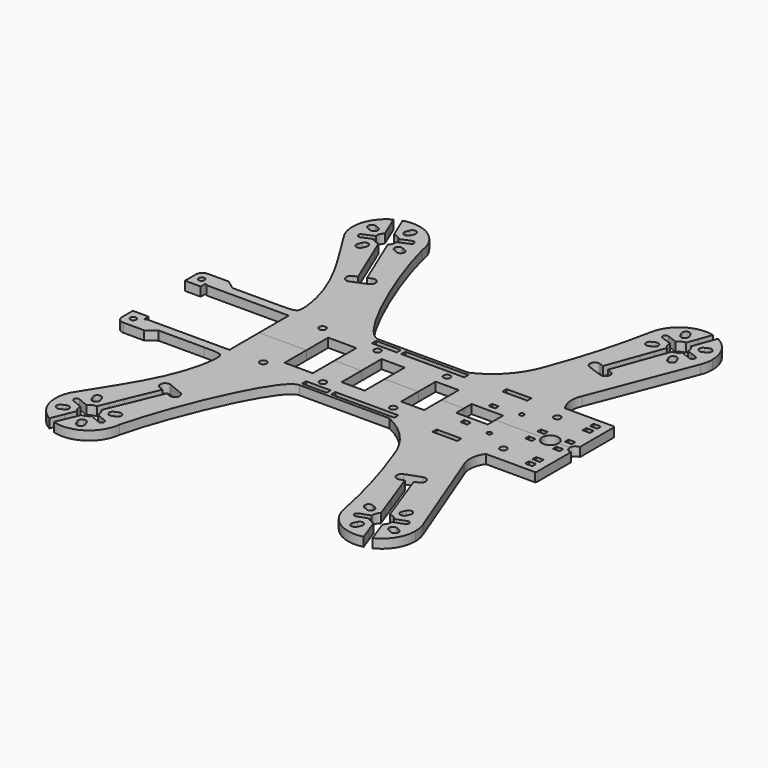
from build123d import *
from build123d import SkipClean  # not in build123d's __all__

# Parameters (mm, degrees)
F0_R     = 1.3067583218
F0_R_2   = 1.5
F0_W     = 11
F0_H     = 2.3
F0_W_2   = 28
F0_W_3   = 3
F0_H_2   = 2
F0_R_3   = 1
F0_W_4   = 7
F0_W_5   = 3.27
F0_H_3   = 1.9745780493
F1_DEPTH = 4


# Not quite as in the source:
# - ends of sketch curves that miss each other by under 0.0002 mm in the source are joined
# - a feature names something its author has since deleted; it is built from what else it names


with BuildPart() as f1:
    # F0 (on Top) → F1 (new body)
    with BuildSketch(Plane.XY):
        with BuildLine():
            Line((23.807834385, 10.9809627828), (66.6183753957, 10.9809627828))
            ThreePointArc((66.6183753957, 10.9809627828), (64.6130521178, 16.2439737053), (65.5746503361, 21.793382168))
            Line((65.5746503361, 21.793382168), (82.7334265347, 66.1261316559))
            ThreePointArc((82.7334265347, 66.1261316559), (75.7149263237, 58.2772137012), (65.2621276006, 57.0107788924))
            Line((65.2621276006, 57.0107788924), (60.1318261331, 42.9153893322))
            Line((60.1318261331, 42.9153893322), (61.889296675, 42.2757224637))
            ThreePointArc((61.889296675, 42.2757224637), (63.1828697728, 39.5016463539), (60.408793663, 38.2080732561))
            Line((60.408793663, 38.2080732561), (53.8309452016, 40.6022139409))
            ThreePointArc((53.8309452016, 40.6022139409), (52.5374310433, 43.3761636546), (55.311380757, 44.6696778129))
            Line((55.311380757, 44.6696778129), (57.0693637919, 44.0301103067))
            Line((57.0693637919, 44.0301103067), (62.1996652593, 58.1254998669))
            ThreePointArc((62.1996652593, 58.1254998669), (55.4315651943, 64.8791097008), (54.1477200077, 74.3538216129))
            ThreePointArc((54.1477200077, 74.3538216129), (49.0043825672, 52.7428496664), (42.0475143877, 31.6456931368))
            ThreePointArc((42.0475143877, 31.6456931368), (35.1236653457, 19.3750412413), (23.807834385, 10.9809627828))
        make_face()
        with BuildLine():
            Line((81.307834385, -10.9840372172), (86.307834385, -10.9840372172))
            ThreePointArc((86.307834385, -10.9840372172), (87.040067432, -9.2162702643), (88.807834385, -8.4840372172))
            Line((88.807834385, -8.4840372172), (88.807834385, 10.2602147337))
            Line((88.807834385, 10.2602147337), (88.807834385, 10.2855553205))
            ThreePointArc((88.807834385, 10.2855553205), (88.6955077799, 10.6869222269), (88.4001219115, 10.9809627828))
            Line((88.4001219115, 10.9809627828), (66.6183753957, 10.9809627828))
            Line((66.6183753957, 10.9809627828), (23.807834385, 10.9809627828))
            Line((23.807834385, 10.9809627828), (-16.192165615, 10.9809627828))
            add(Edge.make_bspline(
                [(-46.3442459805, 73.1007904778), (-41.173171252, 51.9413948059), (-24.192165615, 10.9809627828), (-16.192165615, 10.9809627828)],
                knots=[0, 0, 0, 0, 69.0508576574, 69.0508576574, 69.0508576574, 69.0508576574], degree=3))
            ThreePointArc((-46.3442459805, 73.1007904778), (-46.2810054236, 72.3094979368), (-46.259905361, 71.5159627828))
            ThreePointArc((-46.259905361, 71.5159627828), (-48.3312280894, 63.9285599164), (-53.970550806, 58.4461243811))
            Line((-53.970550806, 58.4461243811), (-48.1929196847, 44.603473673))
            Line((-48.1929196847, 44.603473673), (-46.4646633816, 45.3248114871))
            ThreePointArc((-46.4646633816, 45.3248114871), (-43.6333050022, 44.1609667989), (-44.7971496904, 41.3296084195))
            Line((-44.7971496904, 41.3296084195), (-51.2570532871, 38.6333805908))
            ThreePointArc((-51.2570532871, 38.6333805908), (-54.087935927, 39.7970297238), (-52.9242867941, 42.6279123637))
            Line((-52.9242867941, 42.6279123637), (-51.200432983, 43.3480286655))
            Line((-51.200432983, 43.3480286655), (-56.9780641043, 57.1906793736))
            ThreePointArc((-56.9780641043, 57.1906793736), (-65.7737180803, 57.3039336067), (-72.9794719714, 62.3490764437))
            add(Edge.make_bspline(
                [(-72.9794719714, 62.3490764437), (-63.3735946314, 46.7592850211), (-53.3038261444, 32.6817020671), (-51.3139774001, 14.7110713705)],
                knots=[3.2172773319, 3.2172773319, 3.2172773319, 3.2172773319, 55.6902315894, 55.6902315894, 55.6902315894, 55.6902315894], degree=3))
            add(Edge.make_bspline(
                [(-59.884751521, 9.4825), (-49.8880036175, 9.3324426562), (-51.4223264341, 10.2774120803), (-51.3139774001, 14.7110713705)],
                knots=[0, 0, 0, 0, 10.0397274668, 10.0397274668, 10.0397274668, 10.0397274668], degree=3))
            Line((-59.884751521, 9.4825), (-79.884751521, 9.4825))
            Line((-79.884751521, 9.4825), (-83.984751521, 12.4825))
            Line((-83.984751521, 12.4825), (-93.184751521, 12.4825))
            Line((-93.184751521, 12.4825), (-93.2316647449, 12.4825))
            ThreePointArc((-93.2316647449, 12.4825), (-95.3130075003, 11.6107559793), (-96.184751521, 9.5294132239))
            Line((-96.184751521, 9.5294132239), (-96.184751521, 9.4825))
            Line((-96.184751521, 9.4825), (-96.184751521, 5.4825))
            Line((-96.184751521, 5.4825), (-89.184751521, 5.4825))
            ThreePointArc((-89.184751521, 5.4825), (-88.684751521, 5.9825), (-88.184751521, 5.4825))
            Line((-88.184751521, 5.4825), (-51.684751521, 5.4825))
            Line((-51.684751521, 5.4825), (-51.684751521, -10.9840372172))
            Line((-51.684751521, -10.9840372172), (-30.662165615, -10.9840372172))
            Line((-30.662165615, -10.9840372172), (-30.662165615, 1.1159627828))
            Line((-30.662165615, 1.1159627828), (-18.162165615, 1.1159627828))
            Line((-18.162165615, 1.1159627828), (-18.162165615, -10.9840372172))
            Line((-18.162165615, -10.9840372172), (-6.162165615, -10.9840372172))
            Line((-6.162165615, -10.9840372172), (-6.162165615, 0.1159627828))
            Line((-6.162165615, 0.1159627828), (4.087834385, 0.1159627828))
            Line((4.087834385, 0.1159627828), (4.087834385, -10.9840372172))
            Line((4.087834385, -10.9840372172), (19.087834385, -10.9840372172))
            Line((19.087834385, -10.9840372172), (19.087834385, -1.3840372172))
            Line((19.087834385, -1.3840372172), (29.307834385, -1.3840372172))
            Line((29.307834385, -1.3840372172), (29.307834385, -10.9840372172))
            Line((29.307834385, -10.9840372172), (39.307834385, -10.9840372172))
            Line((39.307834385, -10.9840372172), (39.307834385, -6.7155264844))
            Line((39.307834385, -6.7155264844), (53.307834385, -6.7155264844))
            Line((53.307834385, -6.7155264844), (53.307834385, -10.9840372172))
            Line((53.307834385, -10.9840372172), (74.017834385, -10.9840372172))
            ThreePointArc((74.017834385, -10.9840372172), (77.662834385, -7.3390372172), (81.307834385, -10.9840372172))
        make_face()
        with Locations((-92.384751521, 7.9825)):
            Circle(F0_R, mode=Mode.SUBTRACT)
        with Locations((-36.662165615, 5.4809627828)):
            Circle(F0_R_2, mode=Mode.SUBTRACT)
        with Locations((-11.184751521, 4.1809627828)):
            Circle(F0_R_2, mode=Mode.SUBTRACT)
        with Locations((-10.692165615, 8.4309627828)):
            Rectangle(F0_W, F0_H, mode=Mode.SUBTRACT)
        with Locations((10.807834385, 8.4309627828)):
            Rectangle(F0_W_2, F0_H, mode=Mode.SUBTRACT)
        with Locations((19.807834385, 3.9809627828)):
            Circle(F0_R_2, mode=Mode.SUBTRACT)
        with Locations((46.307834385, -3.2155264844)):
            Rectangle(F0_W_3, F0_H_2, mode=Mode.SUBTRACT)
        with Locations((57.807834385, -2.0190372172)):
            Circle(F0_R_3, mode=Mode.SUBTRACT)
        with Locations((71.517834385, -7.6190372172)):
            Rectangle(F0_W_3, F0_H_2, mode=Mode.SUBTRACT)
        with Locations((83.807834385, -7.6190372172)):
            Rectangle(F0_W_3, F0_H_2, mode=Mode.SUBTRACT)
        with Locations((47.307834385, 8.4309627828)):
            Rectangle(F0_W, F0_H, mode=Mode.SUBTRACT)
        with Locations((68.807834385, 3.9809627828)):
            Circle(F0_R_2, mode=Mode.SUBTRACT)
        Polygon((81.687834385, 5.9782518074), (81.687834385, 8.0809627828), (84.957834385, 8.0809627828), (84.957834385, 5.9782518074), (84.957834385, 4.0036737581), (84.957834385, 1.9009627828), (81.687834385, 1.9009627828), (81.687834385, 4.0036737581), align=None, mode=Mode.SUBTRACT)
        with Locations((-92.684751521, 4.4825)):
            Rectangle(F0_W_4, F0_H_2)
        with BuildLine():
            ThreePointArc((65.2621276006, 57.0107788924), (75.7149263237, 58.2772137012), (82.7334265347, 66.1261316559))
            ThreePointArc((82.7334265347, 66.1261316559), (83.486270311, 68.7744458556), (83.7400946391, 71.5159627828))
            ThreePointArc((83.7400946391, 71.5159627828), (81.4895193699, 79.3993162722), (75.416202451, 84.9063275201))
            Line((75.416202451, 84.9063275201), (73.3649143135, 79.271103595))
            Line((73.3649143135, 79.271103595), (71.6900636377, 74.6700149294))
            ThreePointArc((71.6900636377, 74.6700149294), (72.7174356247, 73.2394210952), (73.0804554083, 71.5159627828))
            ThreePointArc((73.0804554083, 71.5159627828), (73.0780687132, 71.3731720581), (73.0709112943, 71.2305408599))
            Line((73.0709112943, 71.2305408599), (77.6719999599, 69.5556901841))
            ThreePointArc((77.6719999599, 69.5556901841), (78.383174195, 68.0304258767), (76.8579098876, 67.3192516416))
            Line((76.8579098876, 67.3192516416), (72.256821222, 68.9941023174))
            ThreePointArc((72.256821222, 68.9941023174), (70.8217224071, 67.7477343604), (68.9880509133, 67.2471441627))
            Line((68.9880509133, 67.2471441627), (67.3132002375, 62.646055497))
            Line((67.3132002375, 62.646055497), (65.2621276006, 57.0107788924))
        make_face()
        with BuildLine():
            Line((71.6865255454, 61.4383570551), (70.968074214, 62.9790809073))
            ThreePointArc((70.968074214, 62.9790809073), (70.9135396748, 64.2404537845), (71.7658205961, 65.1719325992))
            ThreePointArc((71.7658205961, 65.1719325992), (71.7659371457, 65.1719871288), (71.7660536995, 65.1720416494))
            ThreePointArc((71.7660536995, 65.1720416494), (73.0273231534, 65.2262270051), (73.9585485766, 64.3738448825))
            Line((73.9585485766, 64.3738448825), (74.6936236673, 62.7974712634))
            ThreePointArc((74.6936236673, 62.7974712634), (74.7249665763, 61.5535139642), (73.8793778852, 60.6406109543))
            ThreePointArc((73.8793778852, 60.6406109543), (72.6180046911, 60.5860759997), (71.6865255454, 61.4383570551))
        make_face(mode=Mode.SUBTRACT)
        with BuildLine():
            Line((78.8853157659, 74.3943123226), (77.3445925279, 73.6758612777))
            ThreePointArc((77.3445925279, 73.6758612777), (76.0832108836, 73.6215228577), (75.1518645475, 74.4739489944))
            ThreePointArc((75.1518645475, 74.4739489944), (75.0975261275, 75.7353306387), (75.9499522642, 76.6666769749))
            Line((75.9499522642, 76.6666769749), (77.4906755022, 77.3851280199))
            ThreePointArc((77.4906755022, 77.3851280199), (78.7520571465, 77.4394664398), (79.6834034826, 76.5870403031))
            ThreePointArc((79.6834034826, 76.5870403031), (79.7377419026, 75.3256586588), (78.8853157659, 74.3943123226))
        make_face(mode=Mode.SUBTRACT)
        with BuildLine():
            ThreePointArc((72.35375667, 86.0210939936), (60.7509970609, 84.0881451163), (54.1477200077, 74.3538216129))
            ThreePointArc((54.1477200077, 74.3538216129), (55.4315651943, 64.8791097008), (62.1996652593, 58.1254998669))
            Line((62.1996652593, 58.1254998669), (64.2507544565, 63.7608219705))
            Line((64.2507544565, 63.7608219705), (65.9256051324, 68.3619106361))
            ThreePointArc((65.9256051324, 68.3619106361), (64.8428191889, 69.9241258241), (64.5447574757, 71.8013847056))
            Line((64.5447574757, 71.8013847056), (59.9436688101, 73.4762353814))
            ThreePointArc((59.9436688101, 73.4762353814), (59.232494575, 75.0014996888), (60.7577588824, 75.7126739239))
            Line((60.7577588824, 75.7126739239), (65.358847548, 74.0378232481))
            ThreePointArc((65.358847548, 74.0378232481), (66.7939463629, 75.2841912051), (68.6276178567, 75.7847814029))
            Line((68.6276178567, 75.7847814029), (70.3024685325, 80.3858700685))
            Line((70.3024685325, 80.3858700685), (72.35375667, 86.0210939936))
        make_face()
        with BuildLine():
            ThreePointArc((57.9321409406, 66.4445436419), (57.8778025206, 67.7059252862), (58.7302286573, 68.6372716224))
            Line((58.7302286573, 68.6372716224), (60.2709518953, 69.3557226673))
            ThreePointArc((60.2709518953, 69.3557226673), (61.5323335396, 69.4100610873), (62.4636798757, 68.5576349506))
            ThreePointArc((62.4636798757, 68.5576349506), (62.5180182957, 67.2962533063), (61.665592159, 66.3649069701))
            Line((61.665592159, 66.3649069701), (60.124868921, 65.6464559251))
            ThreePointArc((60.124868921, 65.6464559251), (58.8634872767, 65.5921175051), (57.9321409406, 66.4445436419))
        make_face(mode=Mode.SUBTRACT)
        with BuildLine():
            ThreePointArc((65.8495068393, 77.8601166777), (64.588125195, 77.8057782577), (63.6567788588, 78.6582043944))
            Line((63.6567788588, 78.6582043944), (62.9383275274, 80.1989282467))
            ThreePointArc((62.9383275274, 80.1989282467), (62.8839891074, 81.460309891), (63.7364152441, 82.3916562272))
            ThreePointArc((63.7364152441, 82.3916562272), (64.9977968884, 82.4459946472), (65.9291432246, 81.5935685105))
            Line((65.9291432246, 81.5935685105), (66.6475942696, 80.0528452725))
            ThreePointArc((66.6475942696, 80.0528452725), (66.7019326895, 78.7914636282), (65.8495068393, 77.8601166777))
        make_face(mode=Mode.SUBTRACT)
        with BuildLine():
            ThreePointArc((-46.259905361, 71.5159627828), (-46.2810054236, 72.3094979368), (-46.3442459805, 73.1007904778))
            ThreePointArc((-46.3442459805, 73.1007904778), (-52.8948215222, 83.9307312985), (-65.406740774, 85.8411068492))
            Line((-65.406740774, 85.8411068492), (-63.0964062791, 80.3070408728))
            Line((-63.0964062791, 80.3070408728), (-61.210047547, 75.7885463858))
            ThreePointArc((-61.210047547, 75.7885463858), (-59.355140041, 75.3735044156), (-57.8638020066, 74.1950085268))
            Line((-57.8638020066, 74.1950085268), (-53.3453075196, 76.0813672588))
            ThreePointArc((-53.3453075196, 76.0813672588), (-51.7887128048, 75.4416697569), (-52.4284103068, 73.8850750421))
            Line((-52.4284103068, 73.8850750421), (-56.9469047938, 71.9987163101))
            ThreePointArc((-56.9469047938, 71.9987163101), (-56.9263901261, 71.7577268975), (-56.9195445917, 71.5159627828))
            ThreePointArc((-56.9195445917, 71.5159627828), (-57.2436544819, 69.8836177701), (-58.1668118901, 68.4989236302))
            Line((-58.1668118901, 68.4989236302), (-56.280453158, 63.9804291433))
            Line((-56.280453158, 63.9804291433), (-53.970550806, 58.4461243811))
            ThreePointArc((-53.970550806, 58.4461243811), (-48.3312280894, 63.9285599164), (-46.259905361, 71.5159627828))
        make_face()
        with BuildLine():
            Line((-52.2460218261, 66.0559709047), (-53.816905155, 66.7014730186))
            ThreePointArc((-53.816905155, 66.7014730186), (-54.7130141552, 67.591959671), (-54.7178224889, 68.8552706771))
            ThreePointArc((-54.7178224889, 68.8552706771), (-54.7177737873, 68.8553896293), (-54.7177250764, 68.8555085777))
            ThreePointArc((-54.7177250764, 68.8555085777), (-53.8269435891, 69.7500729149), (-52.5645179851, 69.7543144537))
            Line((-52.5645179851, 69.7543144537), (-50.9557122964, 69.0932294107))
            ThreePointArc((-50.9557122964, 69.0932294107), (-50.0896776729, 68.1996992372), (-50.0928569482, 66.9553512022))
            ThreePointArc((-50.0928569482, 66.9553512022), (-50.9834777453, 66.060458866), (-52.2460218261, 66.0559709047))
        make_face(mode=Mode.SUBTRACT)
        with BuildLine():
            Line((-55.7320326409, 80.4617706639), (-56.3781669556, 78.8893488219))
            ThreePointArc((-56.3781669556, 78.8893488219), (-57.2689272415, 77.9945961026), (-58.5314714596, 77.9903050461))
            ThreePointArc((-58.5314714596, 77.9903050461), (-59.4265939322, 78.8819516537), (-59.4297862468, 80.1453865443))
            Line((-59.4297862468, 80.1453865443), (-58.7843819544, 81.7160318163))
            ThreePointArc((-58.7843819544, 81.7160318163), (-57.8936216684, 82.6107845361), (-56.6310774501, 82.6150755926))
            ThreePointArc((-56.6310774501, 82.6150755926), (-55.7363236975, 81.7243148823), (-55.7320326409, 80.4617706639))
        make_face(mode=Mode.SUBTRACT)
        with BuildLine():
            Line((-66.1038780719, 79.0514964223), (-68.4142125669, 84.5855623986))
            ThreePointArc((-68.4142125669, 84.5855623986), (-75.385470446, 76.1551970159), (-74.7391681393, 65.2349502131))
            add(Edge.make_bspline(
                [(-74.7391681393, 65.2349502131), (-74.1556595147, 64.2664768732), (-73.568437694, 63.3049342425), (-72.9794719714, 62.3490764437)],
                knots=[0, 0, 0, 0, 3.2172773319, 3.2172773319, 3.2172773319, 3.2172773319], degree=3))
            ThreePointArc((-72.9794719714, 62.3490764437), (-65.7737180803, 57.3039336067), (-56.9780641043, 57.1906793736))
            Line((-56.9780641043, 57.1906793736), (-59.2879249509, 62.7248846927))
            Line((-59.2879249509, 62.7248846927), (-61.1742836829, 67.2433791797))
            ThreePointArc((-61.1742836829, 67.2433791797), (-63.029191189, 67.6584211499), (-64.5205292234, 68.8369170388))
            Line((-64.5205292234, 68.8369170388), (-69.0390237104, 66.9505583067))
            ThreePointArc((-69.0390237104, 66.9505583067), (-70.5956184252, 67.5902558086), (-69.9559209232, 69.1468505234))
            Line((-69.9559209232, 69.1468505234), (-65.4374264362, 71.0332092555))
            ThreePointArc((-65.4374264362, 71.0332092555), (-65.2267159208, 72.9222679554), (-64.2175193399, 74.5330019353))
            Line((-64.2175193399, 74.5330019353), (-66.1038780719, 79.0514964223))
        make_face()
        with BuildLine():
            ThreePointArc((-65.7531137168, 60.4165144896), (-66.6478664365, 61.3072747755), (-66.6521574931, 62.5698189939))
            Line((-66.6521574931, 62.5698189939), (-66.0067538091, 64.140465723))
            ThreePointArc((-66.0067538091, 64.140465723), (-65.1161484842, 65.0366235024), (-63.8527186744, 65.0412846117))
            ThreePointArc((-63.8527186744, 65.0412846117), (-62.9579635491, 64.1505245914), (-62.9536718569, 62.8879788578))
            Line((-62.9536718569, 62.8879788578), (-63.5990747037, 61.3173341661))
            ThreePointArc((-63.5990747037, 61.3173341661), (-64.4896798497, 60.4211747742), (-65.7531137168, 60.4165144896))
        make_face(mode=Mode.SUBTRACT)
        with BuildLine():
            ThreePointArc((-67.66743649, 74.1750783521), (-68.5592075259, 73.2810949786), (-69.8219242328, 73.2782018302))
            Line((-69.8219242328, 73.2782018302), (-71.3925701318, 73.9236063802))
            ThreePointArc((-71.3925701318, 73.9236063802), (-72.2873228516, 74.8143666662), (-72.2916139082, 76.0769108845))
            ThreePointArc((-72.2916139082, 76.0769108845), (-71.4008536222, 76.9716636043), (-70.1383094038, 76.9759546609))
            Line((-70.1383094038, 76.9759546609), (-68.5676642623, 76.330550422))
            ThreePointArc((-68.5676642623, 76.330550422), (-67.6715066539, 75.4399461552), (-67.6668442001, 74.1765172175))
            ThreePointArc((-67.6668442001, 74.1765172175), (-67.667139443, 74.1757974148), (-67.66743649, 74.1750783521))
        make_face(mode=Mode.SUBTRACT)
        with Locations((83.322834385, 4.9909627828)):
            Rectangle(F0_W_5, F0_H_3)
    extrude(amount=F1_DEPTH)

    # F2: F1 across face


with BuildPart() as f1_1:
    add(f1.part, clean=False)
    with SkipClean():  # cleaning this boolean's faces spoils the solid; the shape is the same uncleaned
        add(f1.part.mirror(Plane(origin=(83.807834385, -10.9840372172, 2), x_dir=(1, 0, 0), z_dir=(0, -1, 0))), clean=False)


solid = f1_1.part
